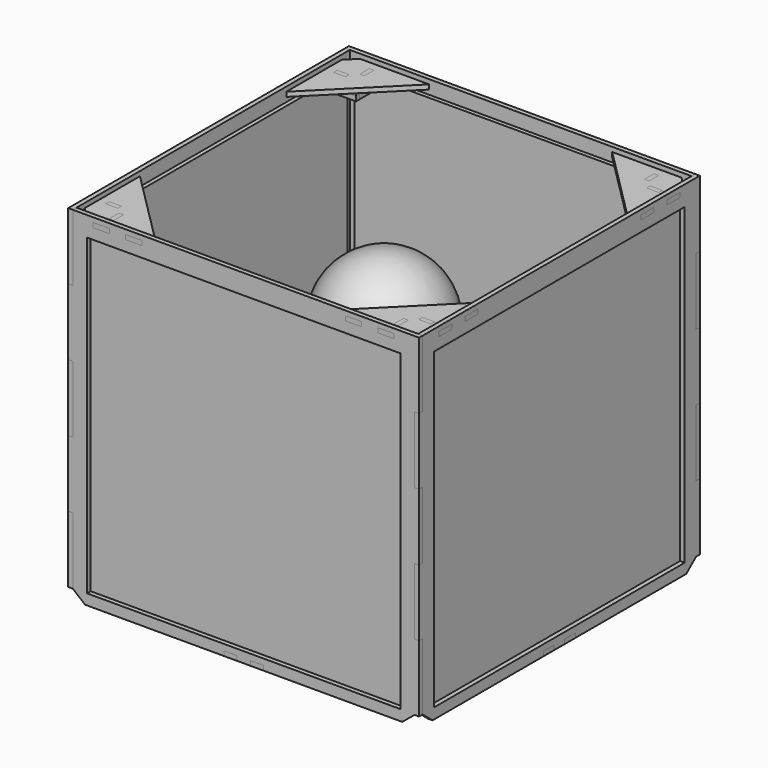
from build123d import *

# Parameters (mm, degrees)
F3_R      = 16
F3_R_2    = 15
F4_DEPTH  = 2.25
F5_W      = 2.25
F5_H      = 6.9285714286
F6_DEPTH  = 38
F7_DEPTH  = 2.25
F8_W      = 2.25
F8_H      = 6.6
F8_W_2    = 6.5
F8_H_2    = 2.25
F9_DEPTH  = 2.25
F11_W     = 160
F11_H     = 160
F12_DEPTH = 2
F13_W     = 154
F13_H     = 154
F13_W_2   = 8
F13_H_2   = 2.25
F14_DEPTH = 2.25
F15_W     = 6
F15_H     = 2.25
F15_W_2   = 2.25
F15_H_2   = 6
F16_DEPTH = 2.25
F18_DEPTH = 2.25
F20_DEPTH = 2.25
F21_W     = 2.25
F21_H     = 6.5
F21_W_2   = 4
F21_H_2   = 2.25
F22_DEPTH = 2.25
F24_DEPTH = 2.25
F25_COUNT = 4


with BuildPart() as f2:
    # F1 (on Front) → F2 (revolve)
    with BuildSketch(Plane.XZ):
        with BuildLine():
            Line((0, 143), (0, 10))
            Line((0, 10), (10, 10))
            Line((10, 10), (11.5, 20))
            Line((11.5, 20), (12.5, 25))
            Line((12.5, 25), (12.5, 36))
            Line((12.5, 36), (16, 36))
            Line((16, 36), (16, 38))
            Line((16, 38), (14, 38))
            Line((14, 38), (14, 40.25))
            Line((14, 40.25), (17.5, 40.25))
            Line((17.5, 40.25), (15, 48.25))
            Line((15, 48.25), (14, 48.25))
            Line((14, 48.25), (14, 63))
            Line((14, 63), (20, 72))
            Line((20, 72), (20, 85))
            Line((20, 85), (24, 95))
            ThreePointArc((24, 95), (26.83281573, 126.416407865), (0, 143))
        make_face()
    revolve(axis=Axis((0, 0, 76.5), (0, 0, -1)))


with BuildPart() as f4:
    # F3 (on face) → F4 (new body)
    with BuildSketch(Plane.XY.offset(38)):
        Polygon((-10.3928571429, 22), (-17.3214285714, 22), (-17.3214285714, 24.25), (-24.25, 24.25), (-24.25, 17.3214285714), (-22, 17.3214285714), (-22, 10.3928571429), (-24.25, 10.3928571429), (-24.25, 3.4642857143), (-22, 3.4642857143), (-22, -3.4642857143), (-24.25, -3.4642857143), (-24.25, -10.3928571429), (-22, -10.3928571429), (-22, -17.3214285714), (-24.25, -17.3214285714), (-24.25, -24.25), (-17.3214285714, -24.25), (-17.3214285714, -22), (-10.3928571429, -22), (-10.3928571429, -24.25), (-3.4642857143, -24.25), (-3.4642857143, -22), (3.4642857143, -22), (3.4642857143, -24.25), (10.3928571429, -24.25), (10.3928571429, -22), (17.3214285714, -22), (17.3214285714, -24.25), (24.25, -24.25), (24.25, -17.3214285714), (22, -17.3214285714), (22, -10.3928571429), (24.25, -10.3928571429), (24.25, -3.4642857143), (22, -3.4642857143), (22, 3.4642857143), (24.25, 3.4642857143), (24.25, 10.3928571429), (22, 10.3928571429), (22, 17.3214285714), (24.25, 17.3214285714), (24.25, 24.25), (17.3214285714, 24.25), (17.3214285714, 22), (10.3928571429, 22), (10.3928571429, 24.25), (3.4642857143, 24.25), (3.4642857143, 22), (-3.4642857143, 22), (-3.4642857143, 24.25), (-10.3928571429, 24.25), align=None)
        Circle(F3_R, mode=Mode.SUBTRACT)
        Circle(F3_R)
        Circle(F3_R_2, mode=Mode.SUBTRACT)
    extrude(amount=F4_DEPTH)


with BuildPart() as f6:
    # F5 (on face) → F6 (new body, through all)
    with BuildSketch(Plane(origin=(0, 0, 38), x_dir=(1, 0, 0), z_dir=(0, 0, -1))):
        with Locations((-23.125, 20.7857142857)):
            Rectangle(F5_W, F5_H)
        with Locations((-23.125, 13.8571428571)):
            Rectangle(F5_W, F5_H)
        with Locations((-23.125, 6.9285714286)):
            Rectangle(F5_W, F5_H)
        with Locations((-23.125, 0)):
            Rectangle(F5_W, F5_H)
        with Locations((-23.125, -6.9285714286)):
            Rectangle(F5_W, F5_H)
        with Locations((-23.125, -13.8571428571)):
            Rectangle(F5_W, F5_H)
        with Locations((-23.125, -20.7857142857)):
            Rectangle(F5_W, F5_H)
    extrude(amount=F6_DEPTH)

    # F5 (on face) → F7 (join, through all)
    with BuildSketch(Plane(origin=(0, 0, 38), x_dir=(1, 0, 0), z_dir=(0, 0, -1))):
        with Locations((-23.125, -13.8571428571)):
            Rectangle(F5_W, F5_H)
        with Locations((-23.125, 0)):
            Rectangle(F5_W, F5_H)
        with Locations((-23.125, 13.8571428571)):
            Rectangle(F5_W, F5_H)
    extrude(amount=-F7_DEPTH)

    # F8 (on face) → F9 (cut, through all)
    with BuildSketch(Plane(origin=(-24.25, 0, 0), x_dir=(0, -1, 0), z_dir=(-1, 0, 0))):
        Polygon((-24.25, 5), (-24.25, 0), (-9.75, 0), (-9.75, 2.25), (-16.25, 2.25), (-16.25, 5), align=None)
        Polygon((9.75, 0), (24.25, 0), (24.25, 5), (24.25, 11.6), (22, 11.6), (22, 5), (16.25, 5), (16.25, 2.25), (9.75, 2.25), align=None)
        with Locations((-23.125, 28.1)):
            Rectangle(F8_W, F8_H)
        with Locations((-23.125, 14.9)):
            Rectangle(F8_W, F8_H)
        with Locations((23.125, 34.7)):
            Rectangle(F8_W, F8_H)
        with Locations((23.125, 21.5)):
            Rectangle(F8_W, F8_H)
        with Locations((0, 1.125)):
            Rectangle(F8_W_2, F8_H_2)
    extrude(amount=-F9_DEPTH, mode=Mode.SUBTRACT)


with BuildPart() as f12:
    # F11 (on offset) → F12 (new body)
    with BuildSketch(Plane.YZ.offset(-82)):
        with Locations((0, 82.25)):
            Rectangle(F11_W, F11_H)
    extrude(amount=-F12_DEPTH)


with BuildPart() as f14:
    # F13 (on face) → F14 (new body)
    with BuildSketch(Plane(origin=(-84, 0, 0), x_dir=(0, -1, 0), z_dir=(-1, 0, 0))):
        Polygon((-84, 136.2), (-86.25, 136.2), (-86.25, 103.4), (-84, 103.4), (-84, 70.6), (-86.25, 70.6), (-86.25, 37.8), (-84, 37.8), (-84, 5), (-78, 0), (-9.75, 0), (-9.75, 2.25), (-3.25, 2.25), (-3.25, 0), (3.25, 0), (3.25, 2.25), (9.75, 2.25), (9.75, 0), (78, 0), (84, 5), (86.25, 5), (86.25, 37.8), (84, 37.8), (84, 70.6), (86.25, 70.6), (86.25, 103.4), (84, 103.4), (84, 136.2), (86.25, 136.2), (86.25, 169), (-84, 169), align=None)
        with Locations((0, 82.25)):
            Rectangle(F13_W, F13_H, mode=Mode.SUBTRACT)
        with Locations((-70, 165.625)):
            Rectangle(F13_W_2, F13_H_2, mode=Mode.SUBTRACT)
        with Locations((-54, 165.625)):
            Rectangle(F13_W_2, F13_H_2, mode=Mode.SUBTRACT)
        with Locations((54, 165.625)):
            Rectangle(F13_W_2, F13_H_2, mode=Mode.SUBTRACT)
        with Locations((70, 165.625)):
            Rectangle(F13_W_2, F13_H_2, mode=Mode.SUBTRACT)
    extrude(amount=F14_DEPTH)


with BuildPart() as f16:
    # F15 (on face) → F16 (new body, through all)
    with BuildSketch(Plane.XY.offset(164.5)):
        Polygon((-84, 74), (-86.25, 74), (-86.25, 66), (-84, 66), (-84, 58), (-86.25, 58), (-86.25, 50), (-84, 50), (-84, 45), (-45, 84), (-50, 84), (-50, 86.25), (-58, 86.25), (-58, 84), (-66, 84), (-66, 86.25), (-74, 86.25), (-74, 84), (-79, 84), (-84, 79), align=None)
        with Locations((-77, 70)):
            Rectangle(F15_W, F15_H, mode=Mode.SUBTRACT)
        with Locations((-70, 77)):
            Rectangle(F15_W_2, F15_H_2, mode=Mode.SUBTRACT)
    extrude(amount=F16_DEPTH)


with BuildPart() as f18:
    # F17 (on face) → F18 (new body, through all)
    with BuildSketch(Plane.XZ.offset(-71.125)):
        Polygon((-74, 166.75), (-80, 166.75), (-80, 164.5), (-82, 164.5), (-82, 157.75), (-68.875, 157.75), (-68.875, 160), (-71.125, 160), (-71.125, 162.25), (-68.875, 162.25), (-68.875, 164.5), (-74, 164.5), align=None)
    extrude(amount=F18_DEPTH)


with BuildPart() as f20:
    # F19 (on face) → F20 (new body, through all)
    with BuildSketch(Plane.YZ.offset(-71.125)):
        Polygon((80, 164.5), (80, 166.75), (74, 166.75), (74, 164.5), (71.125, 164.5), (71.125, 162.25), (68.8749999995, 162.25), (68.8749999995, 160), (71.1249999997, 160), (71.125, 157.75), (82, 157.75), (82, 164.5), align=None)
    extrude(amount=F20_DEPTH)


with BuildPart() as f22:
    # F21 (on Top) → F22 (new body)
    with BuildSketch(Plane.XY):
        Polygon((-22, 16.25), (-84, 16.25), (-84, 9.75), (-86.25, 9.75), (-86.25, 3.25), (-84, 3.25), (-84, -3.25), (-86.25, -3.25), (-86.25, -9.75), (-84, -9.75), (-84, -16.25), (-22, -16.25), (-12.3743686708, -12.3743686708), (-10.2530483272, -10.2530483272), (-8.6620580695, -11.8440385849), (-4.0658639918, -7.2478445072), (-5.6568542495, -5.6568542495), (0, 0), (-5.6568542495, 5.6568542495), (-7.2478445072, 4.0658639918), (-11.8440385849, 8.6620580695), (-10.2530483272, 10.2530483272), (-12.3743686708, 12.3743686708), align=None)
        with Locations((-23.125, -6.5)):
            Rectangle(F21_W, F21_H, mode=Mode.SUBTRACT)
        with Locations((-76, 0)):
            Rectangle(F21_W_2, F21_H_2, mode=Mode.SUBTRACT)
        with Locations((-68, 0)):
            Rectangle(F21_W_2, F21_H_2, mode=Mode.SUBTRACT)
        with Locations((-23.125, 6.5)):
            Rectangle(F21_W, F21_H, mode=Mode.SUBTRACT)
    extrude(amount=F22_DEPTH)


with BuildPart() as f24:
    # F23 (on face) → F24 (new body, through all)
    with BuildSketch(Plane.XZ.offset(-1.125)):
        Polygon((-82, 2.25), (-78, 2.25), (-78, 0), (-74, 0), (-74, 2.25), (-70, 2.25), (-70, 0), (-66, 0), (-66, 2.25), (-62, 2.25), (-62, 6.25), (-82, 6.25), align=None)
    extrude(amount=F24_DEPTH)


with BuildPart() as f25_1:
    # F25: instance of F6
    add(f6.part.rotate(Axis((0, 0, 76.5), (0, 0, -1)), 1 * 360 / F25_COUNT))


with BuildPart() as f25_2:
    # F25: instance of F6
    add(f6.part.rotate(Axis((0, 0, 76.5), (0, 0, -1)), 2 * 360 / F25_COUNT))


with BuildPart() as f25_3:
    # F25: instance of F6
    add(f6.part.rotate(Axis((0, 0, 76.5), (0, 0, -1)), 3 * 360 / F25_COUNT))


with BuildPart() as f25_4:
    # F25: instance of F22
    add(f22.part.rotate(Axis((0, 0, 76.5), (0, 0, -1)), 1 * 360 / F25_COUNT))


with BuildPart() as f25_5:
    # F25: instance of F22
    add(f22.part.rotate(Axis((0, 0, 76.5), (0, 0, -1)), 2 * 360 / F25_COUNT))


with BuildPart() as f25_6:
    # F25: instance of F22
    add(f22.part.rotate(Axis((0, 0, 76.5), (0, 0, -1)), 3 * 360 / F25_COUNT))


with BuildPart() as f25_7:
    # F25: instance of F12
    add(f12.part.rotate(Axis((0, 0, 76.5), (0, 0, -1)), 1 * 360 / F25_COUNT))


with BuildPart() as f25_8:
    # F25: instance of F12
    add(f12.part.rotate(Axis((0, 0, 76.5), (0, 0, -1)), 2 * 360 / F25_COUNT))


with BuildPart() as f25_9:
    # F25: instance of F12
    add(f12.part.rotate(Axis((0, 0, 76.5), (0, 0, -1)), 3 * 360 / F25_COUNT))


with BuildPart() as f25_10:
    # F25: instance of F14
    add(f14.part.rotate(Axis((0, 0, 76.5), (0, 0, -1)), 1 * 360 / F25_COUNT))


with BuildPart() as f25_11:
    # F25: instance of F14
    add(f14.part.rotate(Axis((0, 0, 76.5), (0, 0, -1)), 2 * 360 / F25_COUNT))


with BuildPart() as f25_12:
    # F25: instance of F14
    add(f14.part.rotate(Axis((0, 0, 76.5), (0, 0, -1)), 3 * 360 / F25_COUNT))


with BuildPart() as f25_13:
    # F25: instance of F16
    add(f16.part.rotate(Axis((0, 0, 76.5), (0, 0, -1)), 1 * 360 / F25_COUNT))


with BuildPart() as f25_14:
    # F25: instance of F16
    add(f16.part.rotate(Axis((0, 0, 76.5), (0, 0, -1)), 2 * 360 / F25_COUNT))


with BuildPart() as f25_15:
    # F25: instance of F16
    add(f16.part.rotate(Axis((0, 0, 76.5), (0, 0, -1)), 3 * 360 / F25_COUNT))


with BuildPart() as f25_16:
    # F25: instance of F18
    add(f18.part.rotate(Axis((0, 0, 76.5), (0, 0, -1)), 1 * 360 / F25_COUNT))


with BuildPart() as f25_17:
    # F25: instance of F18
    add(f18.part.rotate(Axis((0, 0, 76.5), (0, 0, -1)), 2 * 360 / F25_COUNT))


with BuildPart() as f25_18:
    # F25: instance of F18
    add(f18.part.rotate(Axis((0, 0, 76.5), (0, 0, -1)), 3 * 360 / F25_COUNT))


with BuildPart() as f25_19:
    # F25: instance of F20
    add(f20.part.rotate(Axis((0, 0, 76.5), (0, 0, -1)), 1 * 360 / F25_COUNT))


with BuildPart() as f25_20:
    # F25: instance of F20
    add(f20.part.rotate(Axis((0, 0, 76.5), (0, 0, -1)), 2 * 360 / F25_COUNT))


with BuildPart() as f25_21:
    # F25: instance of F20
    add(f20.part.rotate(Axis((0, 0, 76.5), (0, 0, -1)), 3 * 360 / F25_COUNT))


with BuildPart() as f25_22:
    # F25: instance of F24
    add(f24.part.rotate(Axis((0, 0, 76.5), (0, 0, -1)), 1 * 360 / F25_COUNT))


with BuildPart() as f25_23:
    # F25: instance of F24
    add(f24.part.rotate(Axis((0, 0, 76.5), (0, 0, -1)), 2 * 360 / F25_COUNT))


with BuildPart() as f25_24:
    # F25: instance of F24
    add(f24.part.rotate(Axis((0, 0, 76.5), (0, 0, -1)), 3 * 360 / F25_COUNT))


solid = Compound([f2.part, f4.part, f6.part, f12.part, f14.part, f16.part, f18.part, f20.part, f22.part, f24.part, f25_1.part, f25_2.part, f25_3.part, f25_4.part, f25_5.part, f25_6.part, f25_7.part, f25_8.part, f25_9.part, f25_10.part, f25_11.part, f25_12.part, f25_13.part, f25_14.part, f25_15.part, f25_16.part, f25_17.part, f25_18.part, f25_19.part, f25_20.part, f25_21.part, f25_22.part, f25_23.part, f25_24.part])
